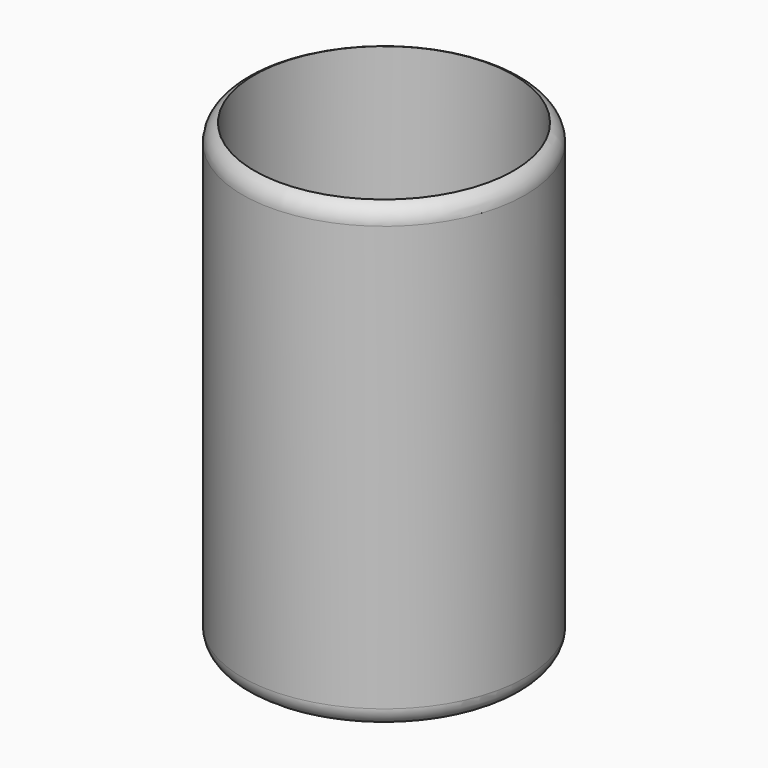
from build123d import *

# Parameters (mm, degrees)
F0_R     = 38.1
F0_R_2   = 34.925
F1_DEPTH = 123.825
F2_DEPTH = 6.35


# Not quite as in the source:
# - a fillet or chamfer that OpenCascade refuses, or shapes differently, is made with other operations: its cross-section is extruded or revolved along the edge and cut away or added


with BuildPart() as f1:
    # F0 (on Top) → F1 (new body)
    with BuildSketch(Plane.XY):
        Circle(F0_R)
        Circle(F0_R_2, mode=Mode.SUBTRACT)
    extrude(amount=F1_DEPTH)

    # F3: fillet of radius 5.08 on 1 edges, made by hand

    # F3_s1 → F3_t2 (revolve, cut)
    with BuildSketch(Plane.XZ):
        with BuildLine():
            ThreePointArc((38.1, 119.1157139607), (37.2321134838, 121.9555202921), (34.925, 123.825))
            Line((34.925, 123.825), (38.1, 123.825))
            Line((38.1, 123.825), (38.1, 119.1157139607))
        make_face()
    revolve(axis=Axis((0, 0, 123.825), (0, 0, 1)), mode=Mode.SUBTRACT)

    # F4: fillet of radius 5.08 on 1 edges, made by hand

    # F4_s1 → F4_t2 (revolve, cut)
    with BuildSketch(Plane.XZ):
        with BuildLine():
            ThreePointArc((38.1, 4.7092860393), (37.2321134838, 1.8694797079), (34.925, 0))
            Line((34.925, 0), (38.1, 0))
            Line((38.1, 0), (38.1, 4.7092860393))
        make_face()
    revolve(axis=Axis((0, 0, 0), (0, 0, 1)), mode=Mode.SUBTRACT)


with BuildPart() as f2:
    # F0 (on Top) → F2 (new body)
    with BuildSketch(Plane.XY):
        Circle(F0_R_2)
    extrude(amount=F2_DEPTH)


solid = Compound([f1.part, f2.part])
